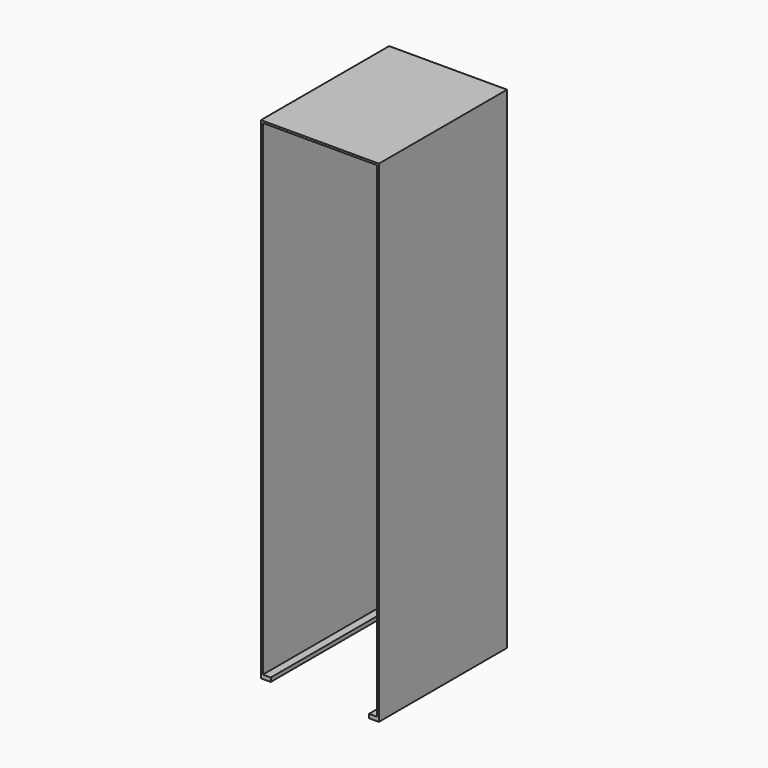
from build123d import *

# Parameters (mm, degrees)
F1_DEPTH = 80
F2_W     = 60
F2_H     = 250
F3_DEPTH = 1.5


# Not quite as in the source:
# - a feature of the source that left no trace in its solid (it failed there, or was rolled back) is left out


with BuildPart() as f1:
    # F0 (on Front) → F1 (new body)
    with BuildSketch(Plane.XZ):
        Polygon((30, 168.8320699929), (-30, 168.8320699929), (-30, -81.1679300071), (-25, -81.1679300071), (-25, -79.1679300071), (-29, -79.1679300071), (-29, 167.8320699929), (29, 167.8320699929), (29, -79.1679300071), (25, -79.1679300071), (25, -81.1679300071), (30, -81.1679300071), align=None)
    extrude(amount=F1_DEPTH)

    # F2 (on face) → F3 (join)
    with BuildSketch(Plane(origin=(0, 0, 0), x_dir=(-1, 0, 0), z_dir=(0, 1, 0))):
        with Locations((0, 43.8320699929)):
            Rectangle(F2_W, F2_H)
    extrude(amount=F3_DEPTH)


solid = f1.part
